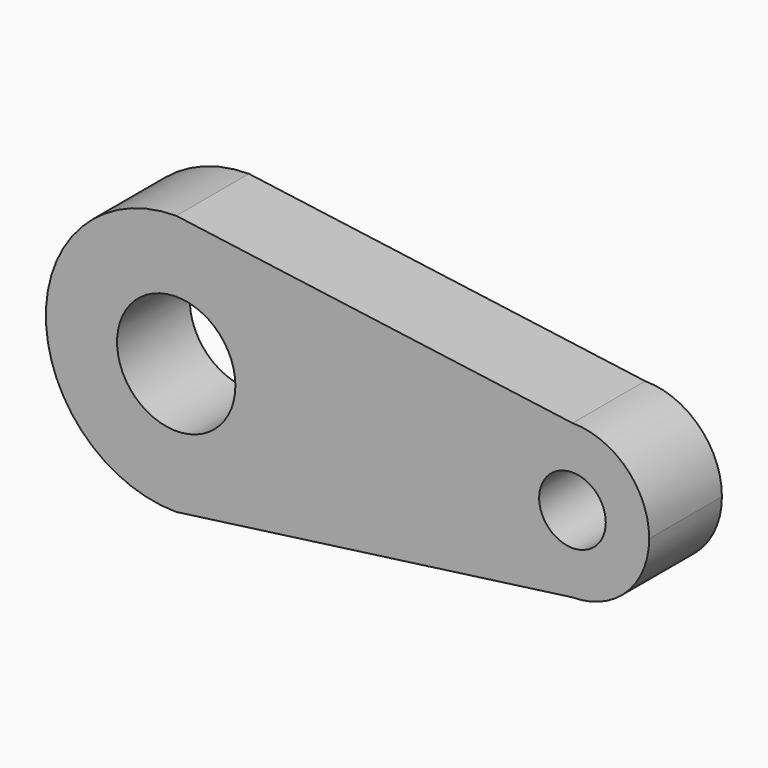
from build123d import *

# Parameters (mm, degrees)
F0_R     = 16.2722693288
F0_R_2   = 9.1584338909
F1_DEPTH = 25


# Not quite as in the source:
# - the program builds the solid bodies; features that only make, move or delete a surface that nothing else refers to are left out


with BuildPart() as f1:
    # F0 (on Front) → F1 (new body)
    with BuildSketch(Plane.XZ):
        with BuildLine():
            Line((-40.7540334754, 34.5627303773), (-50.2872206271, 35.8533678809))
            ThreePointArc((-50.2872206271, 35.8533678809), (-86.140588508, 0), (-50.2872206271, -35.8533678809))
            Line((-50.2872206271, -35.8533678809), (-40.7540334754, -34.5627303773))
            ThreePointArc((-40.7540334754, -34.5627303773), (-21.7630128867, -21.721730161), (-14.4338527462, 0))
            ThreePointArc((-14.4338527462, 0), (-21.7630128867, 21.721730161), (-40.7540334754, 34.5627303773))
        make_face()
        with Locations((-50.2872206271, 0)):
            Circle(F0_R, mode=Mode.SUBTRACT)
        with BuildLine():
            Line((58.6960054934, 21.0988228735), (-40.7540334754, 34.5627303773))
            ThreePointArc((-40.7540334754, 34.5627303773), (-21.7630128867, 21.721730161), (-14.4338527462, 0))
            ThreePointArc((-14.4338527462, 0), (-21.7630128867, -21.721730161), (-40.7540334754, -34.5627303773))
            Line((-40.7540334754, -34.5627303773), (58.6960054934, -21.0988228735))
            ThreePointArc((58.6960054934, -21.0988228735), (37.59718262, 0), (58.6960054934, 21.0988228735))
        make_face()
        with BuildLine():
            ThreePointArc((79.7948283669, 0), (73.6151262223, 14.9191207289), (58.6960054934, 21.0988228735))
            ThreePointArc((58.6960054934, 21.0988228735), (37.59718262, 0), (58.6960054934, -21.0988228735))
            ThreePointArc((58.6960054934, -21.0988228735), (73.6151262223, -14.9191207289), (79.7948283669, 0))
        make_face()
        with Locations((58.6960054934, 0)):
            Circle(F0_R_2, mode=Mode.SUBTRACT)
    extrude(amount=-F1_DEPTH)


solid = f1.part
